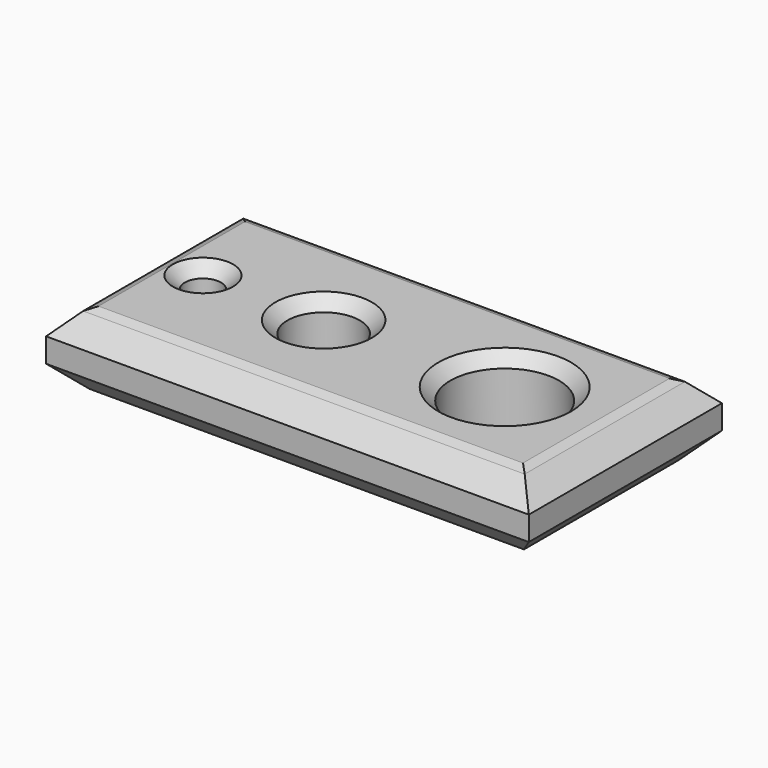
from build123d import *

# Parameters (mm, degrees)
F0_W        = 200
F0_H        = 100
F1_DEPTH    = 15
F2_C1_SIZE  = 10
F2_C2_SIZE  = 10
F2_C3_SIZE  = 10
F2_C4_SIZE  = 10
F2_C5_SIZE  = 10
F2_C6_SIZE  = 10
F2_C7_SIZE  = 10
F2_C8_SIZE  = 10
F3_R        = 15
F3_R_2      = 7.5
F3_R_3      = 22.5
F4_DEPTH    = 30.001
F5_T1_DEPTH = 91.2857086021
F5_T3_DEPTH = 191.2857086021


# Not quite as in the source:
# - a fillet or chamfer that OpenCascade refuses, or shapes differently, is made with other operations: its cross-section is extruded or revolved along the edge and cut away or added


with BuildPart() as f1:
    # F0 (on Top) → F1 (new body, symmetric)
    with BuildSketch(Plane.XY):
        Rectangle(F0_W, F0_H)
    extrude(amount=F1_DEPTH, both=True)

    # F2: chamfer of 10 on 8 edges, made by hand

    # F2_c1
    f2_c1_edges = [f1.edges().sort_by_distance(p)[0] for p in [
        (100, 0, -15),
    ]]
    chamfer(f2_c1_edges, length=F2_C1_SIZE)

    # F2_c2
    f2_c2_edges = [f1.edges().sort_by_distance(p)[0] for p in [
        (100, 0, 15),
    ]]
    chamfer(f2_c2_edges, length=F2_C2_SIZE)

    # F2_c3
    f2_c3_edges = [f1.edges().sort_by_distance(p)[0] for p in [
        (-5, -50, -15),
    ]]
    chamfer(f2_c3_edges, length=F2_C3_SIZE)

    # F2_c4
    f2_c4_edges = [f1.edges().sort_by_distance(p)[0] for p in [
        (-5, -50, 15),
    ]]
    chamfer(f2_c4_edges, length=F2_C4_SIZE)

    # F2_c5
    f2_c5_edges = [f1.edges().sort_by_distance(p)[0] for p in [
        (-100, 5, -15),
    ]]
    chamfer(f2_c5_edges, length=F2_C5_SIZE)

    # F2_c6
    f2_c6_edges = [f1.edges().sort_by_distance(p)[0] for p in [
        (-100, 5, 15),
    ]]
    chamfer(f2_c6_edges, length=F2_C6_SIZE)

    # F2_c7
    f2_c7_edges = [f1.edges().sort_by_distance(p)[0] for p in [
        (0, 50, 15),
    ]]
    chamfer(f2_c7_edges, length=F2_C7_SIZE)

    # F2_c8
    f2_c8_edges = [f1.edges().sort_by_distance(p)[0] for p in [
        (0, 50, -15),
    ]]
    chamfer(f2_c8_edges, length=F2_C8_SIZE)

    # F3 (on face) → F4 (cut, through all)
    with BuildSketch(Plane.XY.offset(15)):
        with Locations((-25, 0)):
            Circle(F3_R)
        with Locations((-75, 0)):
            Circle(F3_R_2)
        with Locations((50, 0)):
            Circle(F3_R_3)
    extrude(amount=-F4_DEPTH, mode=Mode.SUBTRACT)

    # F5: chamfer of 5 on 7 edges, made by hand

    # F5_s2 → F5_t1 (cut)
    with BuildSketch(Plane.XZ.offset(-45.6428543011)):
        Polygon((-91.4644660941, 13.5355339059), (-87.9289321881, 15), (-90, 15), align=None)
        Polygon((91.4644660941, 13.5355339059), (87.9289321881, 15), (90, 15), align=None)
    extrude(amount=F5_T1_DEPTH, mode=Mode.SUBTRACT)

    # F5_s4 → F5_t3 (cut)
    with BuildSketch(Plane.YZ.offset(-95.6428543011)):
        Polygon((41.4644660941, 13.5355339059), (37.9289321881, 15), (40, 15), align=None)
        Polygon((-37.9289321881, 15), (-41.4644660941, 13.5355339059), (-40, 15), align=None)
    extrude(amount=F5_T3_DEPTH, mode=Mode.SUBTRACT)

    # F5_s5 → F5_t6 (revolve, cut)
    with BuildSketch(Plane.XZ):
        Polygon((77.5, 15), (72.5, 10), (72.5, 15), align=None)
    revolve(axis=Axis((50, 0, 15), (0, 0, 1)), mode=Mode.SUBTRACT)

    # F5_s7 → F5_t8 (revolve, cut)
    with BuildSketch(Plane.XZ):
        Polygon((-5, 15), (-10, 10), (-10, 15), align=None)
    revolve(axis=Axis((-25, 0, 15), (0, 0, 1)), mode=Mode.SUBTRACT)

    # F5_s9 → F5_t10 (revolve, cut)
    with BuildSketch(Plane.XZ):
        Polygon((-62.5, 15), (-67.5, 10), (-67.5, 15), align=None)
    revolve(axis=Axis((-75, 0, 15), (0, 0, 1)), mode=Mode.SUBTRACT)


solid = f1.part
